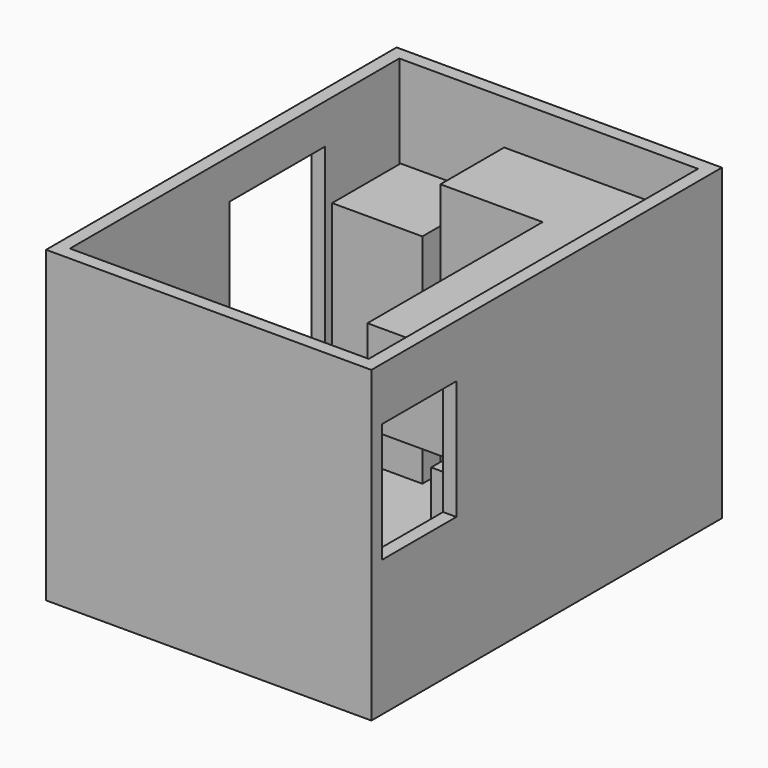
from build123d import *

# Parameters (mm, degrees)
F1_DEPTH  = 2300
F2_W      = 700
F2_H      = 900
F3_DEPTH  = 512.67833
F4_W      = 2450
F4_H      = 3300
F5_DEPTH  = 25
F6_W      = 100
F6_H      = 900
F7_DEPTH  = 300
F8_W      = 680
F8_H      = 645
F9_DEPTH  = 1640
F10_W     = 600
F10_H     = 2400
F11_DEPTH = 800
F13_W     = 600
F13_H     = 1650
F14_DEPTH = 700
F15_W     = 600
F15_H     = 1150
F16_DEPTH = 800
F19_W     = 600
F19_H     = 1350
F20_DEPTH = 800


# Not quite as in the source:
# - a feature of the source that left no trace in its solid (it failed there, or was rolled back) is left out


with BuildPart() as f1:
    # F0 (on Top) → F1 (new body)
    with BuildSketch(Plane.XY):
        Polygon((-1125, 1550), (1125, 1550), (1125, -1550), (-1125, -1550), (-1125, -50), (-1225, -50), (-1225, -1650), (1225, -1650), (1225, 1650), (-1225, 1650), (-1225, 850), (-1125, 850), align=None)
    extrude(amount=F1_DEPTH)

    # F2 (on face) → F3 (cut)
    with BuildSketch(Plane(origin=(1125, 0, 0), x_dir=(0, -1, 0), z_dir=(-1, 0, 0))):
        with Locations((1200, 1450)):
            Rectangle(F2_W, F2_H)
    extrude(amount=-F3_DEPTH, mode=Mode.SUBTRACT)

    # F4 (on face) → F5 (join)
    with BuildSketch(Plane(origin=(0, 0, 0), x_dir=(1, 0, 0), z_dir=(0, 0, -1))):
        Rectangle(F4_W, F4_H)
    extrude(amount=F5_DEPTH)

    # F6 (on face) → F7 (join)
    with BuildSketch(Plane.XY.offset(2300)):
        with Locations((-1175, 400)):
            Rectangle(F6_W, F6_H)
    extrude(amount=-F7_DEPTH)


with BuildPart() as f9:
    # F8 (on face) → F9 (new body)
    with BuildSketch(Plane.XY):
        with Locations((-735, 1177.5)):
            Rectangle(F8_W, F8_H)
    extrude(amount=F9_DEPTH)


with BuildPart() as f11:
    # F10 (on face) → F11 (new body)
    with BuildSketch(Plane.XY):
        Polygon((1075, 1500), (-295, 1500), (-295, 900), (475, 900), (1075, 900), align=None)
        with Locations((775, -300)):
            Rectangle(F10_W, F10_H)
    extrude(amount=F11_DEPTH)

    # F19 (on face) → F20 (cut)
    with BuildSketch(Plane.XY.offset(800)):
        with Locations((775, -825)):
            Rectangle(F19_W, F19_H)
    extrude(amount=-F20_DEPTH, mode=Mode.SUBTRACT)


with BuildPart() as f14:
    # F13 (on offset) → F14 (new body)
    with BuildSketch(Plane.XY.offset(1300)):
        Polygon((1075, 900), (1075, 1500), (-295, 1500), (-295, 900), (475, 900), align=None)
        with Locations((775, 75)):
            Rectangle(F13_W, F13_H)
    extrude(amount=F14_DEPTH)


with BuildPart() as f16:
    # F15 (on face) → F16 (new body)
    with BuildSketch(Plane.XY):
        Polygon((-1075, -150), (-1075, -350), (-475, -350), (-475, -1500), (-469.8359668255, -1500), (-469.8359668255, -150), align=None)
        with Locations((-775, -925)):
            Rectangle(F15_W, F15_H)
    extrude(amount=F16_DEPTH)


solid = Compound([f1.part, f9.part, f11.part, f14.part, f16.part])
